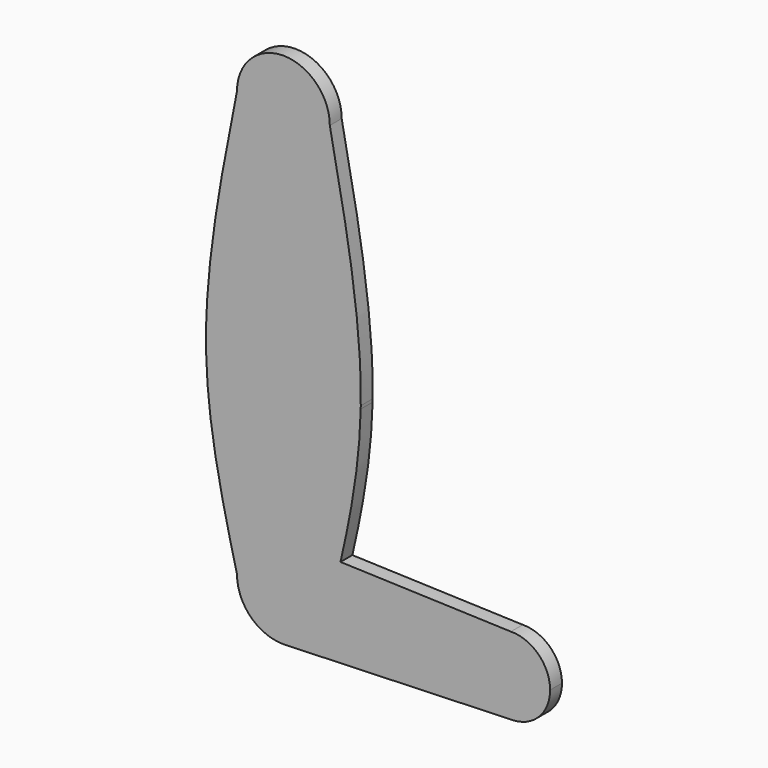
from build123d import *

# Parameters (mm, degrees)
F1_DEPTH = 3.048


with BuildPart() as f1:
    # F0 (on Front) → F1 (new body)
    with BuildSketch(Plane.XZ):
        with BuildLine():
            add(Edge.make_bspline(
                [(0, -29.2028061362), (0.1994290432, -29.2090684708), (0.3988582249, -29.2153378493), (0.5982729839, -29.2216137104)],
                knots=[0, 0, 0, 0, 0.0080246695, 0.0080246695, 0.0080246695, 0.0080246695], degree=3))
            Line((0, -29.2028061362), (0, -38.7278061362))
            Line((0, -38.7278061362), (9.525, -38.7278061362))
            ThreePointArc((9.525, -38.7278061362), (6.9434924632, -32.2075655415), (0.5982729839, -29.2216137104))
        make_face()
        with BuildLine():
            ThreePointArc((-9.525, -38.7278061362), (-6.7351920908, -31.9926140454), (0, -29.2028061362))
            Line((0, -29.2028061362), (0, -15.875))
            ThreePointArc((0, -15.875), (-11.0057082375, -11.4407172498), (-15.8630798211, -0.6150801499))
            add(Edge.make_bspline(
                [(-15.8630798211, -0.6150801499), (-15.5610688303, -14.0326352056), (-12.5430344151, -26.3802206709), (-9.525, -38.7278061362)],
                knots=[0.5347471817, 0.5347471817, 0.5347471817, 0.5347471817, 1, 1, 1, 1], degree=3))
        make_face()
        with BuildLine():
            Line((0, -38.7278061362), (0, -29.2028061362))
            ThreePointArc((0, -29.2028061362), (-6.7351920908, -31.9926140454), (-9.525, -38.7278061362))
            ThreePointArc((-9.525, -38.7278061362), (-6.7351920908, -45.4629982271), (0, -48.2528061362))
            add(Edge.make_bspline(
                [(0, -48.2528061362), (0.2131130588, -48.2456482665), (0.4262259719, -48.2384878681), (0.6393387432, -48.2313250094)],
                knots=[0, 0, 0, 0, 0.6396952306, 0.6396952306, 0.6396952306, 0.6396952306], degree=3))
            ThreePointArc((0.6393387432, -48.2313250094), (6.957561589, -45.2330318614), (9.525, -38.7278061362))
            Line((9.525, -38.7278061362), (0, -38.7278061362))
        make_face()
        with BuildLine():
            Line((0, -15.875), (0, -29.2028061362))
            ThreePointArc((0, -29.2028061362), (0.2992842663, -29.2075091909), (0.5982729839, -29.2216137104))
            add(Edge.make_bspline(
                [(0.5982729839, -29.2216137104), (4.3416181778, -29.339422014), (8.0798811955, -29.4595146085), (11.716745228, -29.5781777813)],
                knots=[0.0080246695, 0.0080246695, 0.0080246695, 0.0080246695, 0.1586610028, 0.1586610028, 0.1586610028, 0.1586610028], degree=3))
            add(Edge.make_bspline(
                [(15.8630798211, -0.6150801499), (15.6355353264, -10.7242843795), (13.866216965, -20.2261112434), (11.7167452282, -29.578177782)],
                knots=[0.5347471817, 0.5347471817, 0.5347471817, 0.5347471817, 0.8852831578, 0.8852831578, 0.8852831578, 0.8852831578], degree=3))
            ThreePointArc((15.8630798211, -0.6150801499), (11.0057082375, -11.4407172498), (0, -15.875))
        make_face()
        with BuildLine():
            ThreePointArc((0.5982729839, -29.2216137104), (0.2992842663, -29.2075091909), (0, -29.2028061362))
            add(Edge.make_bspline(
                [(0, -29.2028061362), (0.1994290432, -29.2090684708), (0.3988582249, -29.2153378493), (0.5982729839, -29.2216137104)],
                knots=[0, 0, 0, 0, 0.0080246695, 0.0080246695, 0.0080246695, 0.0080246695], degree=3))
        make_face()
        with BuildLine():
            ThreePointArc((-15.8630798211, -0.6150801499), (-11.0057082375, -11.4407172498), (0, -15.875))
            Line((0, -15.875), (0, 0))
            Line((0, 0), (0, 15.875))
            ThreePointArc((0, 15.875), (-11.2253201513, 11.2253201513), (-15.875, 0))
            add(Edge.make_bspline(
                [(-15.875, 0), (-15.8716656679, -0.2052784728), (-15.8676890566, -0.4103039216), (-15.8630798211, -0.6150801499)],
                knots=[0.5276465798, 0.5276465798, 0.5276465798, 0.5276465798, 0.5347471817, 0.5347471817, 0.5347471817, 0.5347471817], degree=3))
        make_face()
        with BuildLine():
            Line((0, 0), (0, -15.875))
            ThreePointArc((0, -15.875), (11.0057082375, -11.4407172498), (15.8630798211, -0.6150801499))
            add(Edge.make_bspline(
                [(15.875, 0), (15.8716656679, -0.2052784728), (15.8676890566, -0.4103039216), (15.8630798211, -0.6150801499)],
                knots=[0.5276465798, 0.5276465798, 0.5276465798, 0.5276465798, 0.5347471817, 0.5347471817, 0.5347471817, 0.5347471817], degree=3))
            ThreePointArc((15.875, 0), (11.2253201513, 11.2253201513), (0, 15.875))
            Line((0, 15.875), (0, 0))
        make_face()
        with BuildLine():
            add(Edge.make_bspline(
                [(0.5982729839, -29.2216137104), (4.3416181778, -29.339422014), (8.0798811955, -29.4595146085), (11.716745228, -29.5781777813)],
                knots=[0.0080246695, 0.0080246695, 0.0080246695, 0.0080246695, 0.1586610028, 0.1586610028, 0.1586610028, 0.1586610028], degree=3))
            ThreePointArc((0.5982729839, -29.2216137104), (6.9434924632, -32.2075655415), (9.525, -38.7278061362))
            add(Edge.make_bspline(
                [(11.7167452282, -29.578177782), (11.0133064179, -32.63874678), (10.2691532089, -35.6832764581), (9.525, -38.7278061362)],
                knots=[0.8852831578, 0.8852831578, 0.8852831578, 0.8852831578, 1, 1, 1, 1], degree=3))
        make_face()
        with BuildLine():
            add(Edge.make_bspline(
                [(11.7167452282, -29.578177782), (11.0133064179, -32.63874678), (10.2691532089, -35.6832764581), (9.525, -38.7278061362)],
                knots=[0.8852831578, 0.8852831578, 0.8852831578, 0.8852831578, 1, 1, 1, 1], degree=3))
            Line((9.525, -38.7278061362), (38.8504122414, -38.7278061362))
            ThreePointArc((38.8504122414, -38.7278061362), (41.0703889722, -33.2220061112), (46.4885436218, -30.7959535986))
            add(Edge.make_bspline(
                [(46.6014932618, -30.7924955428), (46.5682462049, -30.7929887265), (46.5283758233, -30.7939133608), (46.4885436218, -30.7959535986)],
                knots=[0.9751953485, 0.9751953485, 0.9751953485, 0.9751953485, 1, 1, 1, 1], degree=3))
            ThreePointArc((46.6014932618, -30.7924955428), (46.6427611197, -30.7916334188), (46.684032903, -30.7909859082))
            add(Edge.make_bspline(
                [(11.716745228, -29.5781777813), (30.5622726651, -30.1930674385), (46.6851234184, -30.7695755158), (46.684032903, -30.7909859082)],
                knots=[0.1586610028, 0.1586610028, 0.1586610028, 0.1586610028, 0.9392294066, 0.9392294066, 0.9392294066, 0.9392294066], degree=3))
        make_face()
        with BuildLine():
            Line((38.8504122414, -38.7278061362), (9.525, -38.7278061362))
            ThreePointArc((9.525, -38.7278061362), (6.957561589, -45.2330318614), (0.6393387432, -48.2313250094))
            add(Edge.make_bspline(
                [(0.6393387432, -48.2313250094), (16.0478252892, -47.7134357647), (31.455570606, -47.182685244), (46.8640654981, -46.6649408164)],
                knots=[0.6396952306, 0.6396952306, 0.6396952306, 0.6396952306, 46.8909606742, 46.8909606742, 46.8909606742, 46.8909606742], degree=3))
            ThreePointArc((46.8640654981, -46.6649408164), (41.2022412981, -44.3673261834), (38.8504122414, -38.7278061362))
        make_face()
        with BuildLine():
            ThreePointArc((-15.875, 0), (-15.8720196755, -0.3075978225), (-15.8630798211, -0.6150801499))
            add(Edge.make_bspline(
                [(-15.875, 0), (-15.8716656679, -0.2052784728), (-15.8676890566, -0.4103039216), (-15.8630798211, -0.6150801499)],
                knots=[0.5276465798, 0.5276465798, 0.5276465798, 0.5276465798, 0.5347471817, 0.5347471817, 0.5347471817, 0.5347471817], degree=3))
        make_face()
        with BuildLine():
            add(Edge.make_bspline(
                [(15.875, 0), (15.8716656679, -0.2052784728), (15.8676890566, -0.4103039216), (15.8630798211, -0.6150801499)],
                knots=[0.5276465798, 0.5276465798, 0.5276465798, 0.5276465798, 0.5347471817, 0.5347471817, 0.5347471817, 0.5347471817], degree=3))
            ThreePointArc((15.8630798211, -0.6150801499), (15.8720196755, -0.3075978225), (15.875, 0))
        make_face()
        with BuildLine():
            add(Edge.make_bspline(
                [(0, -48.2528061362), (0.2131130588, -48.2456482665), (0.4262259719, -48.2384878681), (0.6393387432, -48.2313250094)],
                knots=[0, 0, 0, 0, 0.6396952306, 0.6396952306, 0.6396952306, 0.6396952306], degree=3))
            ThreePointArc((0, -48.2528061362), (0.3198497567, -48.2474343398), (0.6393387432, -48.2313250094))
        make_face()
        with BuildLine():
            ThreePointArc((46.4885436218, -30.7959535986), (41.0703889722, -33.2220061112), (38.8504122414, -38.7278061362))
            ThreePointArc((38.8504122414, -38.7278061362), (41.2022412981, -44.3673261834), (46.8640654981, -46.6649408164))
            add(Edge.make_bspline(
                [(46.8640654981, -46.6649408164), (46.9909147503, -46.6606785252), (47.1177640532, -46.6564171153), (47.2446134078, -46.6521566014)],
                knots=[46.8909606742, 46.8909606742, 46.8909606742, 46.8909606742, 47.2717206688, 47.2717206688, 47.2717206688, 47.2717206688], degree=3))
            ThreePointArc((47.2446134078, -46.6521566014), (52.5597824651, -44.1766060381), (54.7254122414, -38.7278061362))
            ThreePointArc((54.7254122414, -38.7278061362), (52.3637244693, -33.078538551), (46.684032903, -30.7909859082))
            add(Edge.make_bspline(
                [(46.684032903, -30.7909859082), (46.6839826557, -30.7919724263), (46.6497004182, -30.7917804424), (46.6014932618, -30.7924955428)],
                knots=[0.9392294066, 0.9392294066, 0.9392294066, 0.9392294066, 0.9751953485, 0.9751953485, 0.9751953485, 0.9751953485], degree=3))
            ThreePointArc((46.6014932618, -30.7924955428), (46.5450122879, -30.7940235666), (46.4885436218, -30.7959535986))
        make_face()
        with BuildLine():
            ThreePointArc((-15.875, 0), (-11.2253201513, 11.2253201513), (0, 15.875))
            Line((0, 15.875), (0, 39.0321981638))
            ThreePointArc((0, 39.0321981638), (-6.7351920908, 41.822006073), (-9.525, 48.5571981638))
            add(Edge.make_bspline(
                [(-9.525, 48.5571981638), (-12.8238873086, 31.9057330322), (-16.1227746172, 15.2542679006), (-15.875, 0)],
                knots=[0, 0, 0, 0, 0.5276465798, 0.5276465798, 0.5276465798, 0.5276465798], degree=3))
        make_face()
        with BuildLine():
            Line((0, 39.0321981638), (0, 15.875))
            ThreePointArc((0, 15.875), (11.2253201513, 11.2253201513), (15.875, 0))
            add(Edge.make_bspline(
                [(9.525, 48.5571981638), (12.8238873086, 31.9057330322), (16.1227746172, 15.2542679006), (15.875, 0)],
                knots=[0, 0, 0, 0, 0.5276465798, 0.5276465798, 0.5276465798, 0.5276465798], degree=3))
            ThreePointArc((9.525, 48.5571981638), (6.7351920908, 41.822006073), (0, 39.0321981638))
        make_face()
        with BuildLine():
            add(Edge.make_bspline(
                [(46.684032903, -30.7909859082), (46.6839826557, -30.7919724263), (46.6497004182, -30.7917804424), (46.6014932618, -30.7924955428)],
                knots=[0.9392294066, 0.9392294066, 0.9392294066, 0.9392294066, 0.9751953485, 0.9751953485, 0.9751953485, 0.9751953485], degree=3))
            ThreePointArc((46.684032903, -30.7909859082), (46.6427611197, -30.7916334188), (46.6014932618, -30.7924955428))
        make_face()
        with BuildLine():
            add(Edge.make_bspline(
                [(46.6014932618, -30.7924955428), (46.5682462049, -30.7929887265), (46.5283758233, -30.7939133608), (46.4885436218, -30.7959535986)],
                knots=[0.9751953485, 0.9751953485, 0.9751953485, 0.9751953485, 1, 1, 1, 1], degree=3))
            ThreePointArc((46.4885436218, -30.7959535986), (46.5450122879, -30.7940235666), (46.6014932618, -30.7924955428))
        make_face()
        with BuildLine():
            add(Edge.make_bspline(
                [(46.8640654981, -46.6649408164), (46.9909147503, -46.6606785252), (47.1177640532, -46.6564171153), (47.2446134078, -46.6521566014)],
                knots=[46.8909606742, 46.8909606742, 46.8909606742, 46.8909606742, 47.2717206688, 47.2717206688, 47.2717206688, 47.2717206688], degree=3))
            ThreePointArc((46.8640654981, -46.6649408164), (47.0544161215, -46.6608309019), (47.2446134078, -46.6521566014))
        make_face()
        with BuildLine():
            ThreePointArc((-9.525, 48.5571981638), (-6.7351920908, 41.822006073), (0, 39.0321981638))
            ThreePointArc((0, 39.0321981638), (6.7351920908, 41.822006073), (9.525, 48.5571981638))
            ThreePointArc((9.525, 48.5571981638), (0, 58.0821981638), (-9.525, 48.5571981638))
        make_face()
    extrude(amount=F1_DEPTH)


solid = f1.part
